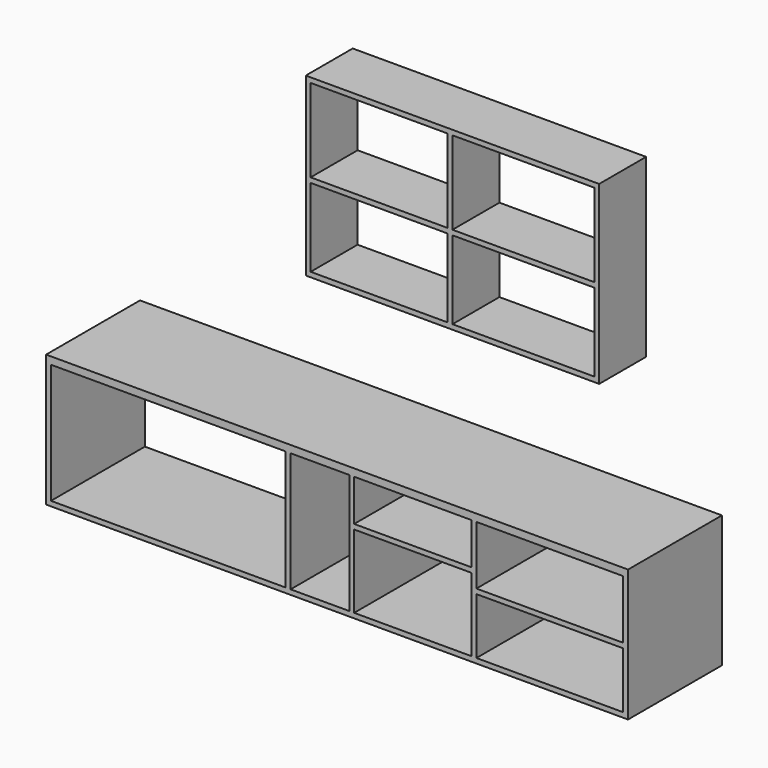
from build123d import *

# Parameters (mm, degrees)
F0_W     = 1524
F0_H     = 914.4
F0_W_2   = 711.2
F0_H_2   = 406.4
F0_H_3   = 431.8
F0_W_3   = 736.6
F2_DEPTH = 304.8
F0_W_4   = 3022.6
F0_H_4   = 685.8
F0_W_5   = 1219.2
F0_H_5   = 622.3
F0_W_6   = 304.8
F0_W_7   = 609.6
F0_H_6   = 381
F0_W_8   = 762
F0_H_7   = 292.1
F0_H_8   = 215.9
F0_H_9   = 304.8
F3_DEPTH = 609.6


# Not quite as in the source:
# - the program builds the solid bodies; features that only make, move or delete a surface that nothing else refers to are left out


with BuildPart() as f2:
    # F0 (on Front) → F2 (new body)
    with BuildSketch(Plane.XZ):
        with Locations((25.4, 271.7650001948)):
            Rectangle(F0_W, F0_H)
        with Locations((-355.6, 43.1650001948)):
            Rectangle(F0_W_2, F0_H_2, mode=Mode.SUBTRACT)
        with Locations((-355.6, 487.6650001948)):
            Rectangle(F0_W_2, F0_H_3, mode=Mode.SUBTRACT)
        with Locations((393.7, 43.1650001948)):
            Rectangle(F0_W_3, F0_H_2, mode=Mode.SUBTRACT)
        with Locations((393.7, 487.6650001948)):
            Rectangle(F0_W_3, F0_H_3, mode=Mode.SUBTRACT)
    extrude(amount=F2_DEPTH)


with BuildPart() as f3:
    # F0 (on Front) → F3 (new body)
    with BuildSketch(Plane.XZ):
        with Locations((-330.2, -1125.2349998052)):
            Rectangle(F0_W_4, F0_H_4)
        with Locations((-1206.5, -1131.5849998052)):
            Rectangle(F0_W_5, F0_H_5, mode=Mode.SUBTRACT)
        with Locations((-419.1, -1131.5849998052)):
            Rectangle(F0_W_6, F0_H_5, mode=Mode.SUBTRACT)
        with Locations((63.5, -1252.2349998052)):
            Rectangle(F0_W_7, F0_H_6, mode=Mode.SUBTRACT)
        with Locations((774.7, -1296.6849998052)):
            Rectangle(F0_W_8, F0_H_7, mode=Mode.SUBTRACT)
        with Locations((63.5, -928.3849998052)):
            Rectangle(F0_W_7, F0_H_8, mode=Mode.SUBTRACT)
        with Locations((774.7, -972.8349998052)):
            Rectangle(F0_W_8, F0_H_9, mode=Mode.SUBTRACT)
    extrude(amount=F3_DEPTH)


solid = Compound([f2.part, f3.part])
